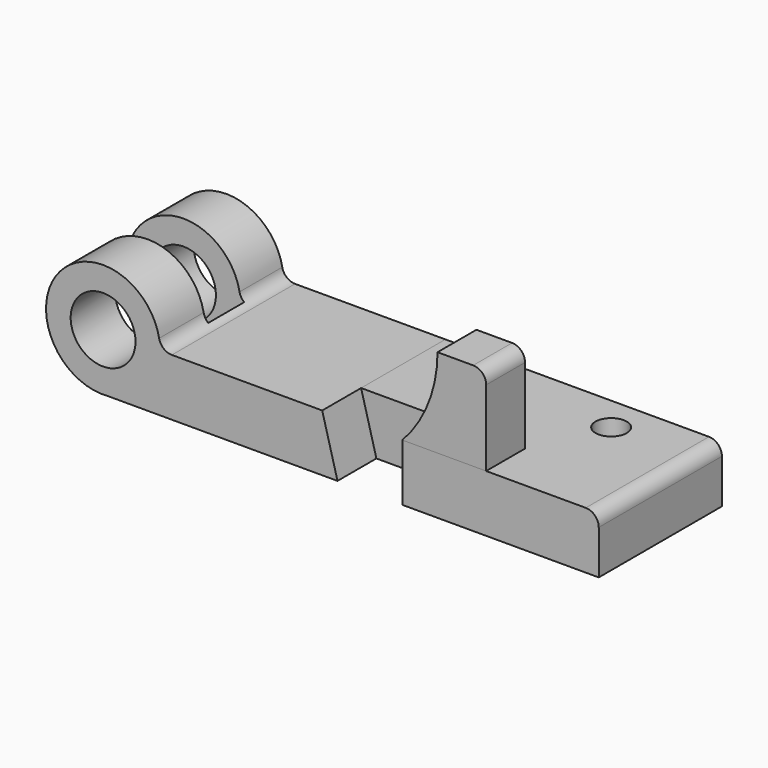
from build123d import *

# Parameters (mm, degrees)
F0_R          = 12.7
F1_DEPTH      = 60.325
F2_DEPTH      = 60.325
F3_DEPTH      = 19.05
F4_DEPTH      = 19.05
F5_W          = 49.9406978488
F5_H          = 17.5811611116
F5_R          = 6.1151869595
F6_DEPTH      = 34.799
F6_DEPTH_BACK = 25.4
F7_R          = 5.0799
F8_R          = 5.08


# Not quite as in the source:
# - a fillet or chamfer is up to 0.001 mm smaller than in the source, because OpenCascade refuses the exact size


with BuildPart() as f1:
    # F0 (on Front) → F1 (new body)
    with BuildSketch(Plane.XZ):
        with BuildLine():
            Line((-21.805210435, 13.050036882), (-85.3053104329, 13.050036882))
            ThreePointArc((-85.3053104329, 13.050036882), (-124.0845666969, 28.1408106558), (-105.929653819, -9.301963118))
            Line((-105.929653819, -9.301963118), (-15.810810435, -9.301963118))
            Line((-15.810810435, -9.301963118), (-21.805210435, 13.050036882))
        make_face()
        with Locations((-107.657210435, 12.9831765975)):
            Circle(F0_R, mode=Mode.SUBTRACT)
    extrude(amount=-F1_DEPTH)


with BuildPart() as f2:
    # F0 (on Front) → F2 (new body)
    with BuildSketch(Plane.XZ):
        Polygon((9.589189565, 13.050036882), (-21.805210435, 13.050036882), (-15.810810435, -9.301963118), (9.589189565, -9.301963118), align=None)
        Polygon((42.431389565, 13.050036882), (9.589189565, 13.050036882), (9.589189565, -9.301963118), (86.551189565, -9.301963118), (86.551189565, 13.050036882), align=None)
    extrude(amount=-F2_DEPTH)

    # F0 (on Front) → F4 (cut)
    with BuildSketch(Plane.XZ):
        Polygon((9.589189565, 13.050036882), (-21.805210435, 13.050036882), (-15.810810435, -9.301963118), (9.589189565, -9.301963118), align=None)
    extrude(amount=-F4_DEPTH, mode=Mode.SUBTRACT)


with BuildPart() as f3:
    # F0 (on Front) → F3 (new body)
    with BuildSketch(Plane.XZ):
        with BuildLine():
            ThreePointArc((23.381389565, 47.848036882), (19.8072049266, 29.1323945161), (9.589189565, 13.050036882))
            Line((9.589189565, 13.050036882), (42.431389565, 13.050036882))
            Line((42.431389565, 13.050036882), (42.431389565, 42.768036882))
            ThreePointArc((42.431389565, 42.768036882), (40.9434920134, 46.3601393304), (37.351389565, 47.848036882))
            Line((37.351389565, 47.848036882), (23.381389565, 47.848036882))
        make_face()
    extrude(amount=-F3_DEPTH)


with BuildPart() as f6_tool:
    # F5 (on face) → F6 (new body, two sides)
    with BuildSketch(Plane.XY.offset(13.050036882)) as f6_sk:
        with Locations((-108.8782735169, 30.5912997574)):
            Rectangle(F5_W, F5_H)
        with Locations((54.1933812201, 46.5162657201)):
            Circle(F5_R)
    extrude(amount=F6_DEPTH)
    extrude(f6_sk.sketch, amount=-F6_DEPTH_BACK)


with BuildPart() as f1_1:
    add(f1.part)

    # F6: cut by f6_tool
    add(f6_tool.part, mode=Mode.SUBTRACT)

    # F7 (radius 5.08 in the source; OpenCascade refuses exactly that, so slightly less here)
    f7_edges = [f1_1.edges().sort_by_distance(p)[0] for p in [
        (-85.30531, 10.90036, 13.050037),
    ]]
    fillet(f7_edges, radius=F7_R)


with BuildPart() as f2_1:
    add(f2.part)

    # F6: cut by f6_tool
    add(f6_tool.part, mode=Mode.SUBTRACT)

    # F8
    f8_edges = [f2_1.edges().sort_by_distance(p)[0] for p in [
        (86.55119, 30.1625, 13.050037),
    ]]
    fillet(f8_edges, radius=F8_R)


solid = Compound([f3.part, f1_1.part, f2_1.part])
